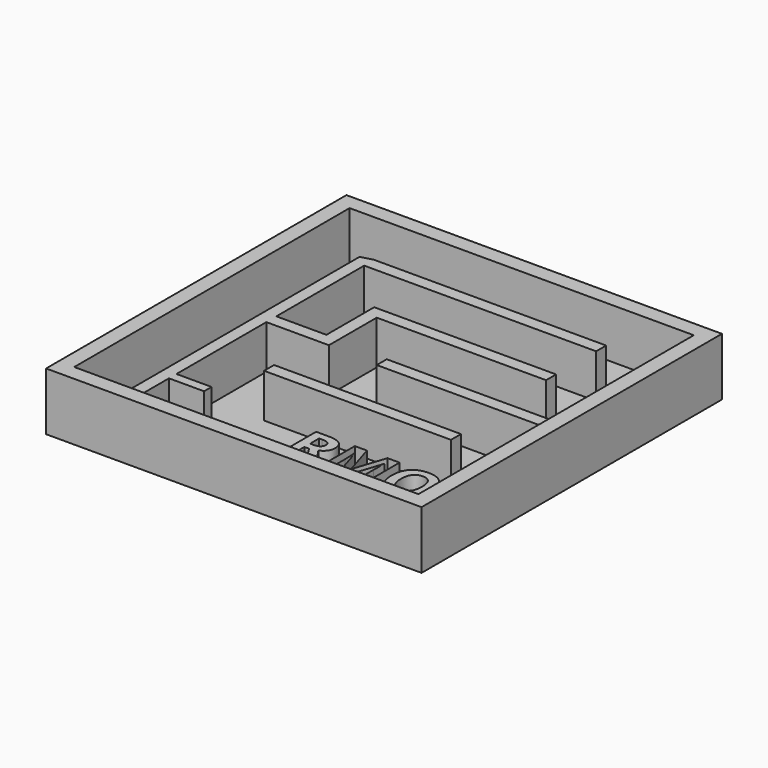
from build123d import *

# Parameters (mm, degrees)
F0_W         = 38.1
F0_H         = 38.1
F1_DEPTH     = 0.79375
F2_W         = 38.1
F2_H         = 38.1
F2_W_2       = 34.925
F2_H_2       = 34.925
F3_DEPTH     = 5.08
F4_W         = 23.5353277876
F4_H         = 1.27
F4_W_2       = 5.08
F4_W_3       = 3.5633865291
F4_H_2       = 0.9510135549
F4_W_4       = 17.1853277876
F4_W_5       = 18.9633277876
F4_TEXT_SIZE = 5.9505898826
F5_DEPTH     = 4.445


# Not quite as in the source:
# - the program builds the solid bodies; features that only make, move or delete a surface that nothing else refers to are left out
# - Text() gives the source's letters only with a copy of the font that has no kerning and outlines rounded to 1/6400 em; it was checked with that copy


with BuildPart() as f1:
    # F0 (on Top) → F1 (new body)
    with BuildSketch(Plane.XY):
        with Locations((-2.1977052093, -2.5823102158)):
            Rectangle(F0_W, F0_H)
    extrude(amount=F1_DEPTH)

    # F2 (on face) → F3 (join)
    with BuildSketch(Plane.XY.offset(0.79375)):
        with Locations((-2.1977052093, -2.5823102158)):
            Rectangle(F2_W, F2_H)
        with Locations((-2.1977052093, -2.5823102158)):
            Rectangle(F2_W_2, F2_H_2, mode=Mode.SUBTRACT)
    extrude(amount=F3_DEPTH)

    # F4 (on face) → F5 (join)
    with BuildSketch(Plane.XY.offset(0.79375)):
        with Locations((-1.582869103, 9.4826897842)):
            Rectangle(F4_W, F4_H)
        with Locations((-10.8105329968, -2.9299963849)):
            Rectangle(F4_W_2, F4_H)
        with Locations((-11.5688397323, -15.4403169932)):
            Rectangle(F4_W_3, F4_H_2)
        Polygon((-8.2705329968, -2.2949963849), (-8.2705329968, -3.5649963849), (-7.0005329968, -3.5649963849), (-7.0005329968, 2.4976897842), (-8.2705329968, 2.4976897842), align=None)
        Polygon((-8.2705329968, 3.7676897842), (-8.2705329968, 2.4976897842), (-7.0005329968, 2.4976897842), (10.1847947907, 2.4976897842), (10.1847947907, 3.7676897842), align=None)
        with Locations((6.672130897, -3.2173102158)):
            Rectangle(F4_W_4, F4_H)
        with Locations((1.211130897, -9.5673102158)):
            Rectangle(F4_W_5, F4_H)
        with Locations((0.9499070044, -20.0448102158)):
            Text('RMO', F4_TEXT_SIZE, font='Open Sans', font_style=FontStyle.BOLD, text_align=(TextAlign.LEFT, TextAlign.BOTTOM))
        Polygon((-14.5802052093, -20.0448102158), (-13.3505329968, -20.0448102158), (-13.3505329968, -15.9158237707), (-13.3505329968, -14.9648102158), (-13.3505329968, -3.5649963849), (-13.3505329968, -2.2949963849), (-13.3505329968, 8.8476897842), (-13.3505329968, 10.1176897842), (-14.5802052093, 9.8001897842), align=None)
    extrude(amount=F5_DEPTH)


solid = f1.part
